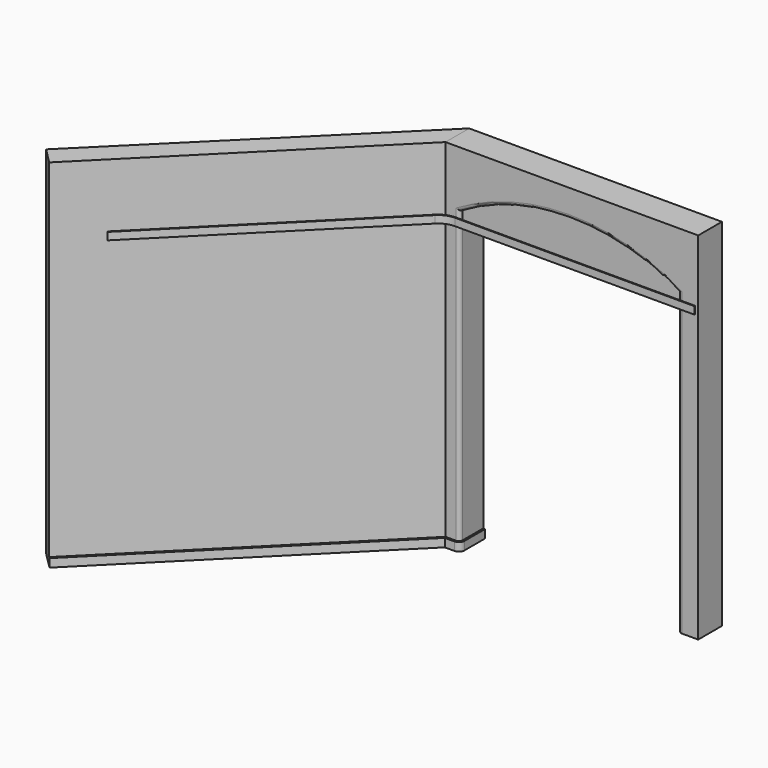
from build123d import *

# Parameters (mm, degrees)
F1_DEPTH  = 101.6
F3_DEPTH  = 177.8
F5_DEPTH  = 25.4
F6_R      = 25.39999
F8_DEPTH  = 2438.4
F10_DEPTH = 57.15
F12_DEPTH = 50.8


# Not quite as in the source:
# - a fillet or chamfer is up to 0.001 mm smaller than in the source, because OpenCascade refuses the exact size
# - ends of sketch curves that miss each other by under 0.0002 mm in the source are joined


with BuildPart() as f1:
    # F0 (on Front) → F1 (new body)
    with BuildSketch(Plane.XZ):
        with BuildLine():
            Line((0, 2049.4625), (0, 1973.2625))
            Line((0, 1973.2625), (1498.6, 1973.2625))
            Line((1498.6, 1973.2625), (1498.6, 2049.4625))
            ThreePointArc((1498.6, 2049.4625), (749.3, 2251.6085390205), (0, 2049.4625))
        make_face()
    extrude(amount=F1_DEPTH)


with BuildPart() as f3:
    # F2 (on face) → F3 (new body)
    with BuildSketch(Plane.XZ.offset(101.6)):
        with BuildLine():
            Line((-96.8375, 0), (0, 0))
            Line((0, 0), (0, 1973.2625))
            Line((0, 1973.2625), (0, 2049.4625))
            ThreePointArc((0, 2049.4625), (749.3, 2251.6085390205), (1498.6, 2049.4625))
            Line((1498.6, 2049.4625), (1498.6, 1973.2625))
            Line((1498.6, 1973.2625), (1498.6, 0))
            Line((1498.6, 0), (1635.125, 0))
            Line((1635.125, 0), (1635.125, 2438.4))
            Line((1635.125, 2438.4), (-96.8375, 2438.4))
            Line((-96.8375, 2438.4), (-96.8375, 0))
        make_face()
    extrude(amount=-F3_DEPTH)

    # F4 (on face) → F5 (join)
    with BuildSketch(Plane.XZ.offset(101.6)):
        with BuildLine():
            Line((-96.8375, 2438.4), (-96.8375, 0))
            Line((-96.8375, 0), (0, 0))
            Line((0, 0), (0, 2049.4625))
            ThreePointArc((0, 2049.4625), (749.3, 2251.6085390205), (1498.6, 2049.4625))
            Line((1498.6, 2049.4625), (1498.6, 0))
            Line((1498.6, 0), (1635.125, 0))
            Line((1635.125, 0), (1635.125, 2438.4))
            Line((1635.125, 2438.4), (-96.8375, 2438.4))
        make_face()
    extrude(amount=F5_DEPTH)

    # F6 (radius 25.4 in the source; OpenCascade refuses exactly that, so slightly less here)
    f6_edges = [f3.edges().sort_by_distance(p)[0] for p in [
        (749.3, -127, 2251.608539),
        (1498.6, -127, 1024.73125),
        (0, -127, 1024.73125),
    ]]
    fillet(f6_edges, radius=F6_R)

    # F9 (on face) → F10 (join)
    with BuildSketch(Plane(origin=(0, 0, 0), x_dir=(1, 0, 0), z_dir=(0, 0, -1))):
        with BuildLine():
            Line((-25.4, 139.7), (-91.5769877579, 139.7))
            Line((-91.5769877579, 139.7), (-1596.5402722185, 1644.6632844607))
            Line((-1596.5402722185, 1644.6632844607), (-1605.5205283396, 1635.6830283396))
            Line((-1605.5205283396, 1635.6830283396), (-96.8375, 127))
            Line((-96.8375, 127), (-20.162967965, 127))
            Line((-20.162967965, 127), (0, 106.837032035))
            Line((0, 106.837032035), (0, -76.2))
            Line((0, -76.2), (12.7, -76.2))
            Line((12.7, -76.2), (12.7, 101.6))
            ThreePointArc((12.7, 101.6), (1.5407683632, 128.5407683632), (-25.4, 139.7))
        make_face()
    extrude(amount=-F10_DEPTH)


with BuildPart() as f8:
    # F7 (on face) → F8 (new body)
    with BuildSketch(Plane.XY.offset(2438.4)):
        Polygon((-1605.5205283396, -1635.6830283396), (-96.8375, -127), (-96.8375, 76.2), (-1713.2836017924, -1527.9199548868), align=None)
    extrude(amount=-F8_DEPTH)


with BuildPart() as f12:
    # F11 (on face) → F12 (new body)
    with BuildSketch(Plane(origin=(0, 0, 1973.2625), x_dir=(1, 0, 0), z_dir=(0, 0, -1))):
        with BuildLine():
            Line((-5.2298163679, 152.4), (1634.5378160477, 152.4))
            Line((1634.5378160477, 152.4), (1634.5378160477, 158.75))
            Line((1634.5378160477, 158.75), (-5.2298163679, 158.75))
            ThreePointArc((-5.2298163679, 158.75), (-61.1207328497, 169.8673914162), (-108.5027639496, 201.5270524183))
            Line((-108.5027639496, 201.5270524183), (-1356.0780931848, 1449.1023860323))
            Line((-1356.0780931848, 1449.1023860323), (-1360.5682212453, 1444.6122579717))
            Line((-1360.5682212453, 1444.6122579717), (-112.9928898208, 197.0369265472))
            ThreePointArc((-112.9928898208, 197.0369265472), (-63.5507714604, 164.0007592453), (-5.2298163679, 152.4))
        make_face()
    extrude(amount=-F12_DEPTH)


solid = Compound([f1.part, f3.part, f8.part, f12.part])
